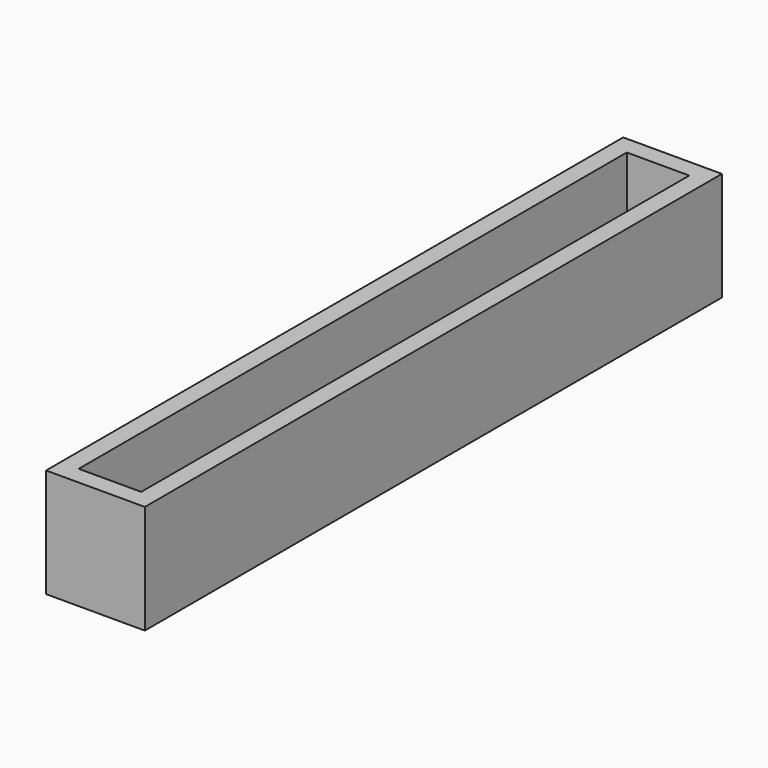
from build123d import *

# Parameters (mm, degrees)
F0_W     = 8.7442658842
F0_H     = 95.895409584
F1_DEPTH = 12.7
F4_T     = 2.54


# Not quite as in the source:
# - the program builds the solid bodies; features that only make, move or delete a surface that nothing else refers to are left out


with BuildPart() as f1:
    # F0 (on Top) → F1 (new body)
    with BuildSketch(Plane.XY):
        with Locations((31.4793456346, -13.4078674018)):
            Rectangle(F0_W, F0_H)
    extrude(amount=F1_DEPTH)

    # F4
    f4_openings = [f1.faces().sort_by_distance(p)[0] for p in [
        (31.479346, -13.407867, 12.7),
    ]]
    offset(amount=F4_T, openings=f4_openings, kind=Kind.INTERSECTION)


solid = f1.part
